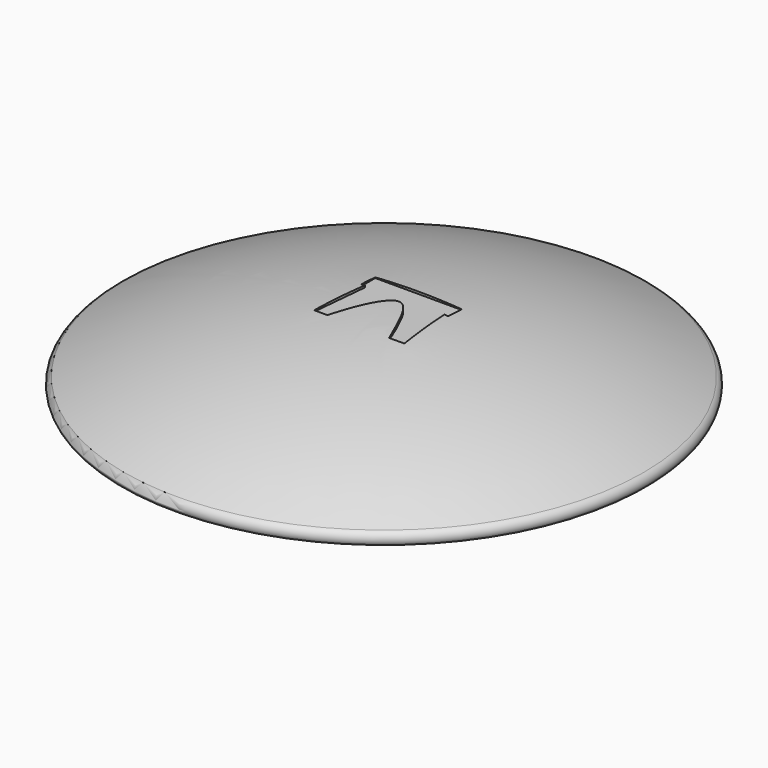
from build123d import *

# Parameters (mm, degrees)
F6_R      = 38.8798944489
F7_DEPTH  = 25.146
F9_DEPTH  = 26.67
F10_W     = 18.4118933976
F10_H     = 2.2933566943
F11_DEPTH = 23.368


# Not quite as in the source:
# - a fillet or chamfer that OpenCascade refuses, or shapes differently, is made with other operations: its cross-section is extruded or revolved along the edge and cut away or added


with BuildPart() as f2:
    # F0 (on Front) → F2 (revolve)
    with BuildSketch(Plane.XZ):
        with BuildLine():
            ThreePointArc((-70.200012, 0), (-35.7013462561, 9.759799439), (0, 13.050012))
            Line((0, 13.050012), (0, 19.05))
            ThreePointArc((0, 19.05), (-39.272581084, 14.215324336), (-76.2, 0))
            Line((-76.2, 0), (-70.200012, 0))
        make_face()
    revolve(axis=Axis((0, 0, 24.1573229432), (0, 0, 1)))

    # F3: fillet of radius 2 on 1 edges, made by hand

    # F3_s1 → F3_t2 (revolve, cut)
    with BuildSketch(Plane.XZ):
        with BuildLine():
            ThreePointArc((-69.7074569816, 3.2775780346), (-70.8242638288, 1.7696123233), (-70.200012, 0))
            Line((-70.200012, 0), (-76.2, 0))
            ThreePointArc((-76.2, 0), (-72.9721325586, 1.6752455717), (-69.7074569816, 3.2775780346))
        make_face()
    revolve(axis=Axis((0, 0, 0), (0, 0, 1)), mode=Mode.SUBTRACT)

    # F6 (on offset) → F7 (cut)
    with BuildSketch(Plane.XY.offset(13.0556)):
        Circle(F6_R)
        with BuildLine():
            ThreePointArc((25.4, 0.3187083348), (25.2716745644, -2.231284746), (24.8879949046, -4.7555117659))
            ThreePointArc((24.8879949046, -4.7555117659), (24.4197271347, -6.6696338625), (23.8044800528, -8.5416939933))
            ThreePointArc((23.8044800528, -8.5416939933), (-24.9979378484, 4.8201640248), (25.4, 0.3187083348))
        make_face(mode=Mode.SUBTRACT)
        with BuildLine():
            Line((0, 0.3187083348), (0, 19.3497721271))
            ThreePointArc((0, 19.3497721271), (-19.0310637922, 0.3187083348), (0, -18.7123554574))
            Line((0, -18.7123554574), (0, 0.3187083348))
        make_face()
        with BuildLine():
            Line((0, 19.3497721271), (0, 19.3687083348))
            ThreePointArc((0, 19.3687083348), (13.2989496278, 13.9533806489), (19.0390180892, 0.7913348654))
            ThreePointArc((19.0390180892, 0.7913348654), (19.9506333706, 0.3253641448), (20.8212014385, -0.2134144487))
            ThreePointArc((20.8212014385, -0.2134144487), (20.8263002903, 0.0526252288), (20.828, 0.3187083348))
            ThreePointArc((20.828, 0.3187083348), (-20.7308721477, 2.3278185842), (20.4403944696, -3.6807738728))
            ThreePointArc((20.4403944696, -3.6807738728), (19.6537458396, -3.1118600746), (18.8168844801, -2.6197807703))
            ThreePointArc((18.8168844801, -2.6197807703), (12.3848096584, -14.1516820769), (0, -18.7312916652))
            Line((0, -18.7312916652), (0, -18.7123554574))
            ThreePointArc((0, -18.7123554574), (-19.0310637922, 0.3187083348), (0, 19.3497721271))
        make_face()
        with BuildLine():
            ThreePointArc((0.0092738827, 19.3497698675), (0.0046369415, 19.3497715622), (0, 19.3497721271))
            Line((0, 19.3497721271), (0, 0.3187083348))
            Line((0, 0.3187083348), (0, -18.7123554574))
            ThreePointArc((0, -18.7123554574), (0.0046369415, -18.7123548925), (0.0092738827, -18.7123531978))
            ThreePointArc((0.0092738827, -18.7123531978), (4.4162974191, 0.3187083348), (0.0092738827, 19.3497698675))
        make_face()
        with BuildLine():
            ThreePointArc((13.1388957402, 1.9248430338), (13.7609973094, 1.9418144736), (14.3831748206, 1.9279027252))
            ThreePointArc((14.3831748206, 1.9279027252), (12.1419924656, 8.1965372147), (7.3325286529, 12.7995508523))
            ThreePointArc((7.3325286529, 12.7995508523), (8.9882975444, 0.3187083348), (7.3325286529, -12.1621341826))
            ThreePointArc((7.3325286529, -12.1621341826), (12.0996579985, -7.6240165515), (14.3651267069, -1.4443980064))
            ThreePointArc((14.3651267069, -1.4443980064), (13.9524158986, -1.4394824186), (13.5398409591, -1.4511569053))
            ThreePointArc((13.5398409591, -1.4511569053), (9.5797965511, -0.2096564514), (13.1388957402, 1.9248430338))
        make_face()
    extrude(amount=-F7_DEPTH, mode=Mode.SUBTRACT)

    # F8 (on offset) → F9 (cut)
    with BuildSketch(Plane.XY.offset(18.034)):
        Polygon((-11.6335004568, 11.633916758), (-11.6335004568, 10.6838271022), (0, 10.6838271022), (11.6335004568, 10.6838271022), (11.6335004568, 11.633916758), align=None)
        Polygon((0, 10.6838271022), (-11.6335004568, 10.6838271022), (-11.6335004568, 7.7160974033), (-10.5779496953, 7.7160974033), (-8.4452219732, 7.7160974033), (-7.4719206453, 7.7160974033), (-6.7395351815, 7.7160974033), (0, 7.7160974033), align=None)
        Polygon((11.6335004568, 10.6838271022), (0, 10.6838271022), (0, 7.7160974033), (6.7395351815, 7.7160974033), (7.4719206453, 7.7160974033), (8.4452219732, 7.7160974033), (10.5779496953, 7.7160974033), (11.6335004568, 7.7160974033), align=None)
        Polygon((-10.5779496953, 7.7160974033), (-11.6335004568, 7.7160974033), (-11.6335004568, 7.0042582229), (-10.6457086273, 7.0042582229), align=None)
        Polygon((-8.4452219732, 7.7160974033), (-10.5779496953, 7.7160974033), (-10.6457086273, 7.0042582229), (-8.5129809052, 7.0042582229), align=None)
        Polygon((11.6335004568, 7.0042582229), (11.6335004568, 7.7160974033), (10.5779496953, 7.7160974033), (10.6457086273, 7.0042582229), align=None)
        Polygon((-8.5129809052, 7.0042582229), (-10.6457086273, 7.0042582229), (-11.6335004568, -3.3729556017), (-12.100125514, -8.275069438), (-9.9865486123, -8.4762577367), align=None)
        Polygon((-8.2961780285, -8.637161644), (-6.8072941135, 7.0042582229), (-7.5396795774, 7.0042582229), (-9.0219870399, -8.5680729442), align=None)
        with BuildLine():
            Line((6.8072941135, 7.0042582229), (-6.8072941135, 7.0042582229))
            Line((-6.8072941135, 7.0042582229), (-8.2961780285, -8.637161644))
            add(Edge.make_bspline(
                [(-8.2961780285, -8.637161644), (-5.5307853524, -1.8041071938), (0, 11.8620017068), (5.5307853524, -1.8041071938), (8.2961780285, -8.637161644)],
                knots=[0, 0, 0, 0, 0.5, 1, 1, 1, 1], degree=3))
            Line((8.2961780285, -8.637161644), (6.8072941135, 7.0042582229))
        make_face()
        Polygon((7.5396795774, 7.0042582229), (6.8072941135, 7.0042582229), (8.2961780285, -8.637161644), (9.0219870399, -8.5680729442), align=None)
        Polygon((10.6457086273, 7.0042582229), (10.5779496953, 7.7160974033), (8.4452219732, 7.7160974033), (8.5129809052, 7.0042582229), align=None)
        Polygon((-7.5396795774, 7.0042582229), (-8.5129809052, 7.0042582229), (-9.9865486123, -8.4762577367), (-9.0219870399, -8.5680729442), align=None)
        Polygon((8.5129809052, 7.0042582229), (7.5396795774, 7.0042582229), (9.0219870399, -8.5680729442), (9.9865486123, -8.4762577367), align=None)
        Polygon((11.6335004568, -3.3729556017), (10.6457086273, 7.0042582229), (8.5129809052, 7.0042582229), (9.9865486123, -8.4762577367), (12.100125514, -8.275069438), align=None)
    extrude(amount=F9_DEPTH, mode=Mode.SUBTRACT)

    # F10 (on offset) → F11 (cut)
    with BuildSketch(Plane.XY.offset(18.034)):
        with Locations((-0.0296542421, 7.2142141871)):
            Rectangle(F10_W, F10_H)
    extrude(amount=F11_DEPTH, mode=Mode.SUBTRACT)


solid = f2.part
